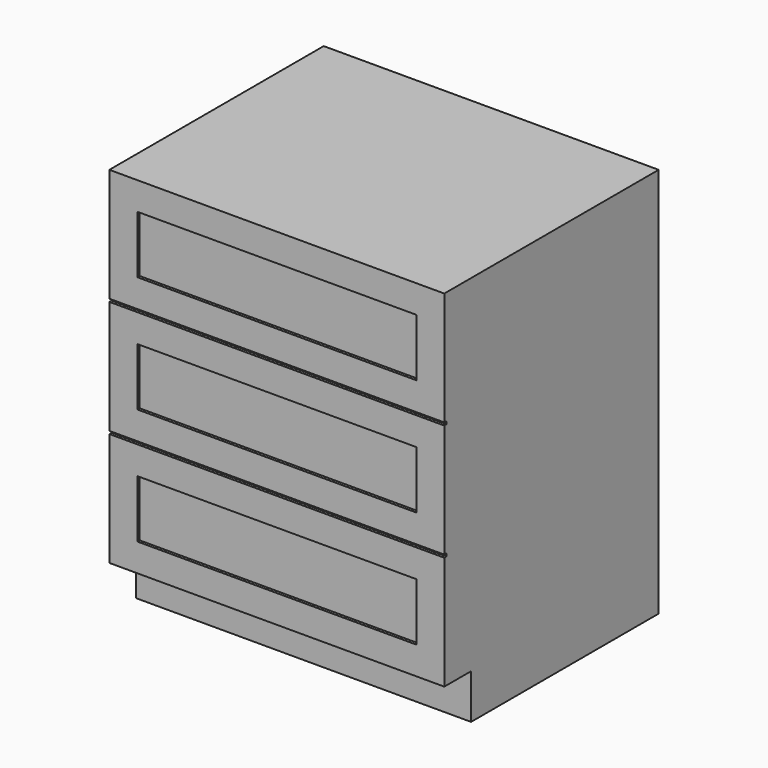
from build123d import *

# Parameters (mm, degrees)
F0_W     = 762
F0_H     = 101.6
F0_H_2   = 258.16306
F0_W_2   = 635
F0_H_3   = 131.16306
F0_H_4   = 3.175
F0_H_5   = 65.47612
F0_H_6   = 65.68694
F1_DEPTH = 609.6
F2_DEPTH = 6.35
F3_DEPTH = 76.2


# Not quite as in the source:
# - a feature names something its author has since deleted; it is built from what else it names


with BuildPart() as f1:
    # F0 (on Front) → F1 (new body)
    with BuildSketch(Plane.XZ):
        with Locations((261.2652602196, -51.4053403184)):
            Rectangle(F0_W, F0_H)
        with Locations((261.2652602196, 128.4761896816)):
            Rectangle(F0_W, F0_H_2)
        with Locations((261.2652602196, 128.4761896816)):
            Rectangle(F0_W_2, F0_H_3, mode=Mode.SUBTRACT)
        with Locations((261.2652602196, 259.1452196816)):
            Rectangle(F0_W, F0_H_4)
        with Locations((261.2652602196, 262.3202196816)):
            Rectangle(F0_W, F0_H_4)
        Polygon((-119.7347397804, 263.9077196816), (642.2652602196, 263.9077196816), (642.2652602196, 393.0946596816), (578.7652602196, 393.0946596816), (578.7652602196, 327.4077196816), (-56.2347397804, 327.4077196816), (-56.2347397804, 393.0946596816), (-119.7347397804, 393.0946596816), align=None)
        Polygon((578.7652602196, 393.0946596816), (642.2652602196, 393.0946596816), (642.2652602196, 522.2815996816), (-119.7347397804, 522.2815996816), (-119.7347397804, 393.0946596816), (-56.2347397804, 393.0946596816), (-56.2347397804, 458.5707796816), (578.7652602196, 458.5707796816), align=None)
        with Locations((261.2652602196, 523.8690996816)):
            Rectangle(F0_W, F0_H_4)
        with Locations((261.2652602196, 527.0440996816)):
            Rectangle(F0_W, F0_H_4)
        with Locations((261.2652602196, 657.7131296816)):
            Rectangle(F0_W, F0_H_2)
        with Locations((261.2652602196, 657.9239496816)):
            Rectangle(F0_W_2, F0_H_3, mode=Mode.SUBTRACT)
        with Locations((261.2652602196, 657.9239496816)):
            Rectangle(F0_W_2, F0_H_3)
        with Locations((261.2652602196, 425.8327196816)):
            Rectangle(F0_W_2, F0_H_5)
        with Locations((261.2652602196, 360.2511896816)):
            Rectangle(F0_W_2, F0_H_6)
        with Locations((261.2652602196, 128.4761896816)):
            Rectangle(F0_W_2, F0_H_3)
    extrude(amount=-F1_DEPTH)

    # F0 (on Front) → F2 (cut)
    with BuildSketch(Plane.XZ):
        with Locations((261.2652602196, 657.9239496816)):
            Rectangle(F0_W_2, F0_H_3)
        with Locations((261.2652602196, 425.8327196816)):
            Rectangle(F0_W_2, F0_H_5)
        with Locations((261.2652602196, 360.2511896816)):
            Rectangle(F0_W_2, F0_H_6)
        with Locations((261.2652602196, 128.4761896816)):
            Rectangle(F0_W_2, F0_H_3)
        with Locations((261.2652602196, 262.3202196816)):
            Rectangle(F0_W, F0_H_4)
        with Locations((261.2652602196, 259.1452196816)):
            Rectangle(F0_W, F0_H_4)
        with Locations((261.2652602196, 527.0440996816)):
            Rectangle(F0_W, F0_H_4)
        with Locations((261.2652602196, 523.8690996816)):
            Rectangle(F0_W, F0_H_4)
    extrude(amount=-F2_DEPTH, mode=Mode.SUBTRACT)

    # F0 (on Front) → F3 (cut)
    with BuildSketch(Plane.XZ):
        with Locations((261.2652602196, -51.4053403184)):
            Rectangle(F0_W, F0_H)
    extrude(amount=-F3_DEPTH, mode=Mode.SUBTRACT)


solid = f1.part
